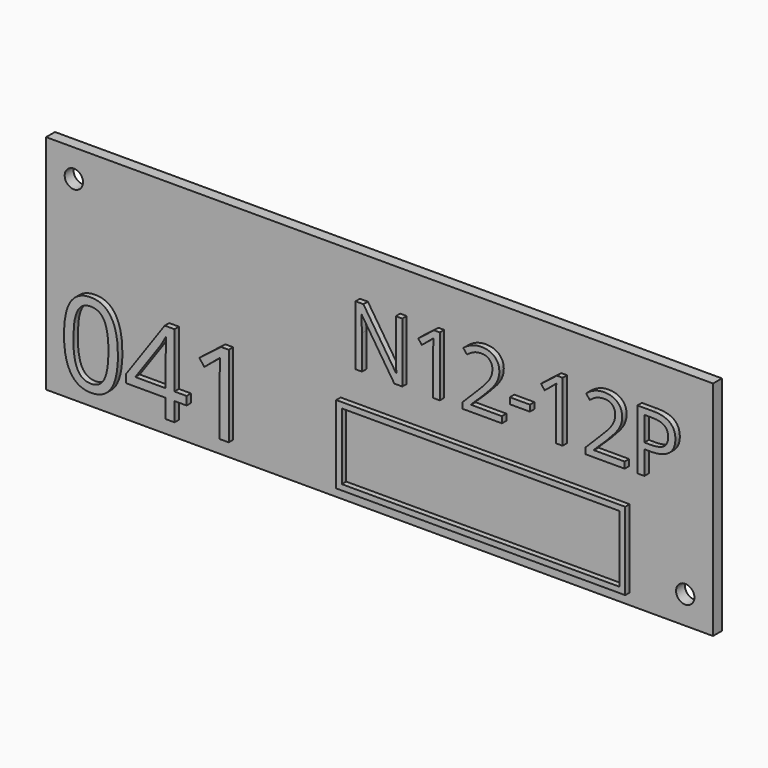
from build123d import *

# Parameters (mm, degrees)
F0_W         = 120
F0_H         = 40
F1_DEPTH     = 2
F3_D         = 3.3
F4_TEXT_SIZE = 15.0824823252
F5_DEPTH     = 1
F6_TEXT_SIZE = 20.5478077656
F7_DEPTH     = 1
F8_W         = 52
F8_H         = 14
F8_W_2       = 49.99999962
F8_H_2       = 11.99999962
F9_DEPTH     = 1


# Not quite as in the source:
# - Text() gives the source's letters only with a copy of the font that has no kerning and outlines rounded to 1/6400 em; it was checked with that copy


with BuildPart() as f1:
    # F0 (on Front) → F1 (new body)
    with BuildSketch(Plane.XZ):
        Rectangle(F0_W, F0_H)
    extrude(amount=F1_DEPTH)

    # F3 (through all)
    with Locations(Plane.XZ.offset(2)):
        with Locations((-55, 15), (55, -15)):
            Hole(F3_D / 2)

    # F4 (on face) → F5 (join)
    with BuildSketch(Plane.XZ.offset(2)):
        with Locations((-5, 2)):
            Text('N12-12P', F4_TEXT_SIZE, font='Open Sans', text_align=(TextAlign.LEFT, TextAlign.BOTTOM))
    extrude(amount=F5_DEPTH)

    # F6 (on face) → F7 (join)
    with BuildSketch(Plane.XZ.offset(2)):
        with Locations((-57, -17)):
            Text('041', F6_TEXT_SIZE, font='Open Sans', text_align=(TextAlign.LEFT, TextAlign.BOTTOM))
    extrude(amount=F7_DEPTH)

    # F8 (on face) → F9 (join)
    with BuildSketch(Plane.XZ.offset(2)):
        with Locations((19, -11)):
            Rectangle(F8_W, F8_H)
        with Locations((19, -11)):
            Rectangle(F8_W_2, F8_H_2, mode=Mode.SUBTRACT)
    extrude(amount=F9_DEPTH)


solid = f1.part
